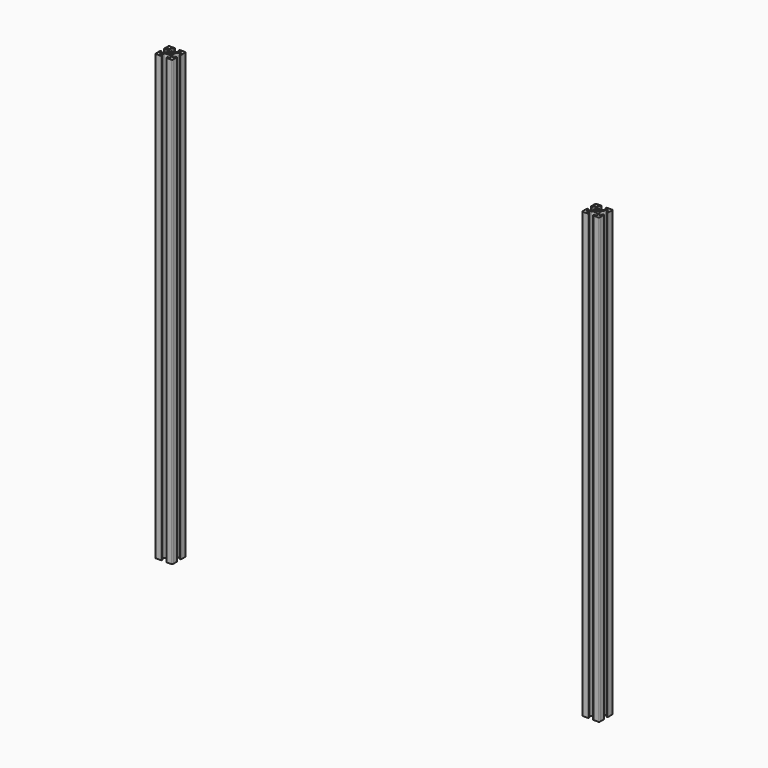
from build123d import *

# Parameters (mm, degrees)
F0_R     = 2.6035
F1_DEPTH = 660.4
F2_R     = 1.18109
F3_R     = 5.08
F4_R     = 0.762
F5_R     = 1.27


# Not quite as in the source:
# - a fillet or chamfer is up to 0.001 mm smaller than in the source, because OpenCascade refuses the exact size


with BuildPart() as f1:
    # F0 (on Top) → F1 (new body)
    with BuildSketch(Plane.XY):
        Polygon((12.7, 3.2385), (12.7, 12.7), (3.2385, 12.7), (3.2385, 10.3378), (8.7752354349, 10.3378), (2.9459354349, 4.5085), (-2.9459354349, 4.5085), (-8.7752354349, 10.3378), (-3.2385, 10.3378), (-3.2385, 12.7), (-12.7, 12.7), (-12.7, 3.2385), (-10.3378, 3.2385), (-10.3378, 8.7752354349), (-4.5085, 2.9459354349), (-4.5085, -2.9459354349), (-10.3378, -8.7752354349), (-10.3378, -3.2385), (-12.7, -3.2385), (-12.7, -12.7), (-3.2385, -12.7), (-3.2385, -10.3378), (-8.7752354349, -10.3378), (-2.9459354349, -4.5085), (2.9459354349, -4.5085), (8.7752354349, -10.3378), (3.2385, -10.3378), (3.2385, -12.7), (12.7, -12.7), (12.7, -3.2385), (10.3378, -3.2385), (10.3378, -8.7752354349), (4.5085, -2.9459354349), (4.5085, 2.9459354349), (10.3378, 8.7752354349), (10.3378, 3.2385), align=None)
        Circle(F0_R, mode=Mode.SUBTRACT)
    extrude(amount=F1_DEPTH)

    # F2 (radius 1.1811 in the source; OpenCascade refuses exactly that, so slightly less here)
    f2_edges = [f1.edges().sort_by_distance(p)[0] for p in [
        (3.2385, 12.7, 330.2),
        (3.2385, 10.3378, 330.2),
        (-3.2385, 12.7, 330.2),
        (-12.7, 3.2385, 330.2),
        (-3.2385, 10.3378, 330.2),
        (-10.3378, 3.2385, 330.2),
        (12.7, 3.2385, 330.2),
        (10.3378, 3.2385, 330.2),
        (12.7, -3.2385, 330.2),
        (10.3378, -3.2385, 330.2),
        (3.2385, -10.3378, 330.2),
        (-3.2385, -10.3378, 330.2),
        (-10.3378, -3.2385, 330.2),
        (-12.7, -3.2385, 330.2),
        (-3.2385, -12.7, 330.2),
        (3.2385, -12.7, 330.2),
    ]]
    fillet(f2_edges, radius=F2_R)

    # F3
    f3_edges = [f1.edges().sort_by_distance(p)[0] for p in [
        (2.945935, 4.5085, 330.2),
        (-2.945935, 4.5085, 330.2),
        (4.5085, -2.945935, 330.2),
        (4.5085, 2.945935, 330.2),
        (2.945935, -4.5085, 330.2),
        (-2.945935, -4.5085, 330.2),
        (-4.5085, -2.945935, 330.2),
        (-4.5085, 2.945935, 330.2),
    ]]
    fillet(f3_edges, radius=F3_R)

    # F4
    f4_edges = [f1.edges().sort_by_distance(p)[0] for p in [
        (8.775235, 10.3378, 330.2),
        (-8.775235, 10.3378, 330.2),
        (-10.3378, 8.775235, 330.2),
        (-10.3378, -8.775235, 330.2),
        (-8.775235, -10.3378, 330.2),
        (8.775235, -10.3378, 330.2),
        (10.3378, -8.775235, 330.2),
        (10.3378, 8.775235, 330.2),
    ]]
    fillet(f4_edges, radius=F4_R)

    # F5
    f5_edges = [f1.edges().sort_by_distance(p)[0] for p in [
        (-12.7, -12.7, 330.2),
        (12.7, -12.7, 330.2),
        (12.7, 12.7, 330.2),
        (-12.7, 12.7, 330.2),
    ]]
    fillet(f5_edges, radius=F5_R)


with BuildPart() as f6_1:
    # F6: copy of F1
    add(f1.part.moved(Location((635, 0, 0))))


solid = Compound([f1.part, f6_1.part])
